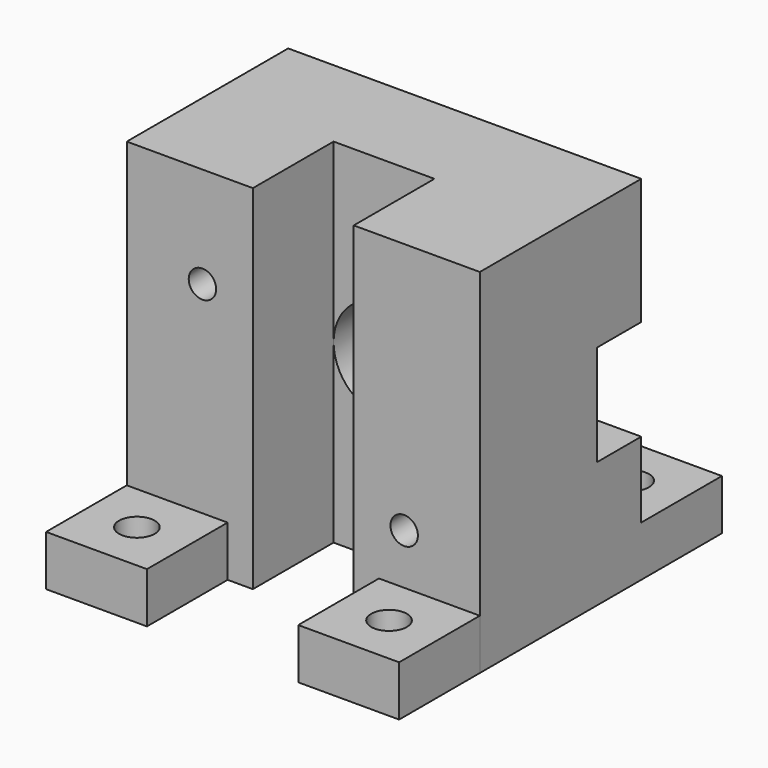
from build123d import *
from build123d import SkipClean  # not in build123d's __all__

# Parameters (mm, degrees)
F0_W             = 44.45
F0_H             = 25.4
F1_DEPTH         = 44.45
F2_W             = 12.7
F2_H             = 44.45
F3_DEPTH         = 12.7
F4_W             = 44.45
F4_H             = 12.7
F5_DEPTH         = 6.985
F7_D             = 12.7
F8_W             = 12.7
F8_H             = 6.35
F9_DEPTH         = 12.7
F9_COPIES2_COUNT = 2
F9_COPIES2_PITCH = 49.595085
F11_D            = 4.4958
F13_D            = 3.4544


# Not quite as in the source:
# - after a boolean that leaves OpenCascade's solid faulty, fix() repairs it
# - a length typed as a fraction of an inch, garbled in the dataset ("3 / 203.2 mm" for 3/8 in), is restored
# - a pattern or mirror of a feature is missing from the dataset's text; its kind, count and spacing are read off the source's solid


with BuildPart() as f1:
    # F0 (on Top) → F1 (new body)
    with BuildSketch(Plane.XY):
        Rectangle(F0_W, F0_H)
    extrude(amount=F1_DEPTH)

    # F2 (on face) → F3 (cut)
    with BuildSketch(Plane.XZ.offset(12.7)):
        with Locations((0, 22.225)):
            Rectangle(F2_W, F2_H)
    extrude(amount=-F3_DEPTH, mode=Mode.SUBTRACT)

    # F4 (on face) → F5 (cut)
    with BuildSketch(Plane(origin=(0, 12.7, 0), x_dir=(-1, 0, 0), z_dir=(0, 1, 0))):
        with Locations((0, 22.225)):
            Rectangle(F4_W, F4_H)
    extrude(amount=-F5_DEPTH, mode=Mode.SUBTRACT)

    # F7 (through all)
    with Locations(Plane.XZ.offset(12.7)):
        with Locations((0, 22.225)):
            Hole(F7_D / 2)

    # F8 (on face) → F9 (join)
    with BuildSketch(Plane(origin=(0, 12.7, 0), x_dir=(-1, 0, 0), z_dir=(0, 1, 0))):
        with Locations((15.875, 3.175)):
            Rectangle(F8_W, F8_H)
    f9 = extrude(amount=F9_DEPTH)

    # F9_copies: F9 across plane
    add(f9.mirror(Plane(origin=(0, 0, 0), x_dir=(0, 0, -1), z_dir=(0, -1, 0))), clean=False)

    # F9_copies1: F9 across plane
    add(f9.mirror(Plane(origin=(0, 0, 0), x_dir=(0, 0, 1), z_dir=(1, 0, 0))), clean=False)

    # F9_copies2: F9 ×2
    with SkipClean():  # cleaning this boolean's faces spoils the solid; the shape is the same uncleaned
        with Locations(*[Vector(0.6401843997, -0.7682212796, 0) * (i * F9_COPIES2_PITCH) for i in range(1, F9_COPIES2_COUNT)]):
            add(f9, clean=False)

    # F11 (through all)
    with Locations(Plane.XY.offset(6.35)):
        with Locations((-15.875, 19.05)):
            f11 = Hole(F11_D / 2)

    add(f1.part.fix(), mode=Mode.REPLACE)

    # F11_copies: F11 across plane
    add(f11.mirror(Plane(origin=(0, 0, 0), x_dir=(0, 0, -1), z_dir=(0, -1, 0))), clean=False, mode=Mode.SUBTRACT)

    # F11_copies1: F11 across plane
    add(f11.mirror(Plane(origin=(0, 0, 0), x_dir=(0, 0, 1), z_dir=(1, 0, 0))), clean=False, mode=Mode.SUBTRACT)

    # F11_copies2: F11 across plane
    add(f11.mirror(Plane(origin=(0, 0, 0), x_dir=(-0.7682212796, -0.6401843997, 0), z_dir=(0.6401843997, -0.7682212796, 0))), clean=False, mode=Mode.SUBTRACT)

    # F13 (through all)
    with Locations(Plane.XZ.offset(12.7)):
        with Locations((-12.7, 31.75), (12.7, 12.7)):
            Hole(F13_D / 2)


solid = f1.part
